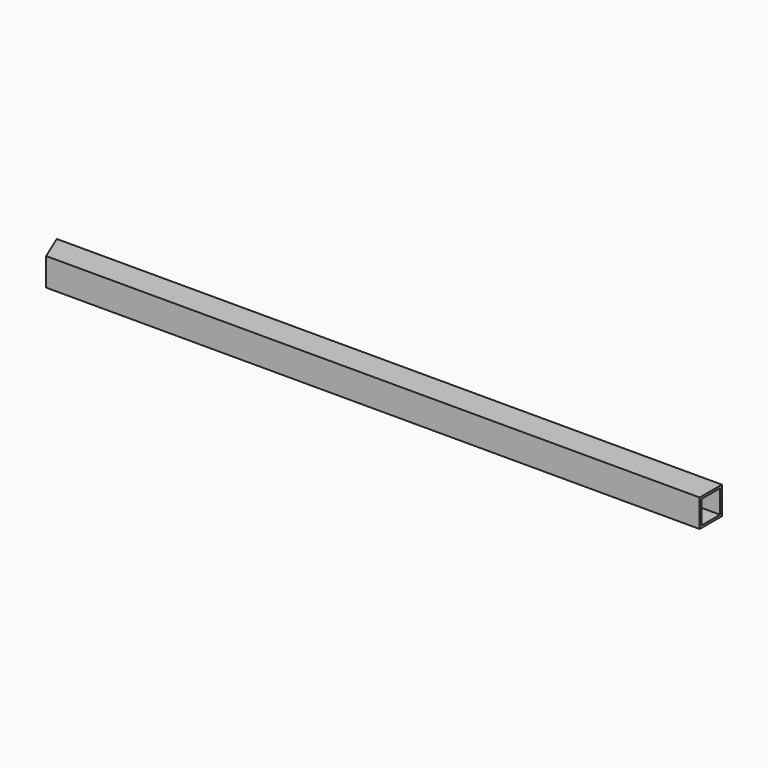
from build123d import *

# Parameters (mm, degrees)
F0_W        = 25
F0_H        = 25
F0_W_2      = 21
F0_H_2      = 21
F1_DEPTH    = 600
F2_T1_DEPTH = 180.5602235744


# Not quite as in the source:
# - a fillet or chamfer that OpenCascade refuses, or shapes differently, is made with other operations: its cross-section is extruded or revolved along the edge and cut away or added


with BuildPart() as f1:
    # F0 (on Right) → F1 (new body)
    with BuildSketch(Plane.YZ):
        Rectangle(F0_W, F0_H)
        Rectangle(F0_W_2, F0_H_2, mode=Mode.SUBTRACT)
    extrude(amount=F1_DEPTH)

    # F2: chamfer of 30 x 12.4264068712 on 1 edges, made by hand

    # F2_s2 → F2_t1 (cut)
    with BuildSketch(Plane.XY.offset(-90.2801117872)):
        Polygon((12.4264068712, -12.5), (0, 17.5), (0, -12.5), align=None)
    extrude(amount=F2_T1_DEPTH, mode=Mode.SUBTRACT)


solid = f1.part
